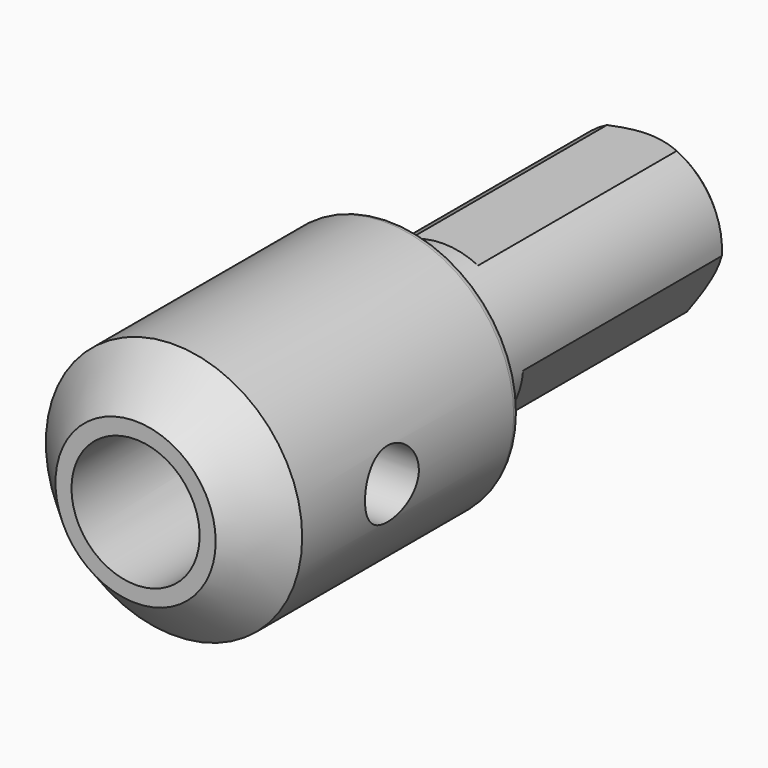
from build123d import *

# Parameters (mm, degrees)
F0_R            = 8
F1_DEPTH        = 20
F2_R            = 5
F3_DEPTH        = 20
F5_DEPTH        = 16
F5_COPIES_COUNT = 3
F6_SIZE         = 0.49999
F7_R            = 0.5
F9_D            = 8
F9_DEPTH        = 18
F9_TIP          = 2.4034424761
F10_R           = 2.1
F11_DEPTH       = 8.25
F12_SIZE        = 3


# Not quite as in the source:
# - a fillet or chamfer is up to 0.001 mm smaller than in the source, because OpenCascade refuses the exact size
# - a pattern or mirror of a feature is missing from the dataset's text; its kind, count and spacing are read off the source's solid


with BuildPart() as f1:
    # F0 (on Front) → F1 (new body)
    with BuildSketch(Plane.XZ):
        Circle(F0_R)
    extrude(amount=-F1_DEPTH)

    # F2 (on face) → F3 (join)
    with BuildSketch(Plane(origin=(0, 20, 0), x_dir=(-1, 0, 0), z_dir=(0, 1, 0))):
        Circle(F2_R)
    extrude(amount=F3_DEPTH)

    # F4 (on face) → F5 (cut)
    with BuildSketch(Plane(origin=(0, 40, 0), x_dir=(-1, 0, 0), z_dir=(0, 1, 0))):
        with BuildLine():
            ThreePointArc((2.1794494718, 4.5), (0, 5), (-2.1794494718, 4.5))
            Line((-2.1794494718, 4.5), (2.1794494718, 4.5))
        make_face()
    f5 = extrude(amount=-F5_DEPTH, mode=Mode.SUBTRACT)

    # F5_copies: F5 ×3 about axis
    f5_copies_axis = Axis((0, 0, 0), (0, 1, 0))
    for i in range(1, F5_COPIES_COUNT):
        add(f5.rotate(f5_copies_axis, i * 360 / F5_COPIES_COUNT), mode=Mode.SUBTRACT)

    # F6 (size 0.5 in the source; OpenCascade refuses exactly that, so slightly less here)
    f6_edges = [f1.edges().sort_by_distance(p)[0] for p in [
        (4.330127, 40, 2.5),
        (-4.996709, 40, -0.18139),
        (0, 40, -5),
        (-4.236582, 40, 2.655443),
    ]]
    chamfer(f6_edges, length=F6_SIZE)

    # F7
    f7_edges = [f1.edges().sort_by_distance(p)[0] for p in [
        (-8, 20, 0),
        (5, 20, 0),
    ]]
    fillet(f7_edges, radius=F7_R)

    # F9
    with Locations(Plane.XZ):
        with Locations((0, 0)):
            Hole(F9_D / 2, depth=F9_DEPTH)
            with Locations((0, 0, -(F9_DEPTH + F9_TIP / 2))):  # 118° drill point
                Cone(0, F9_D / 2, F9_TIP, mode=Mode.SUBTRACT)

    # F10 (on Right) → F11 (cut, symmetric)
    with BuildSketch(Plane.YZ):
        with Locations((10, 0)):
            Circle(F10_R)
    extrude(amount=F11_DEPTH, both=True, mode=Mode.SUBTRACT)

    # F12
    f12_edges = [f1.edges().sort_by_distance(p)[0] for p in [
        (-8, 0, 0),
    ]]
    chamfer(f12_edges, length=F12_SIZE)


solid = f1.part
